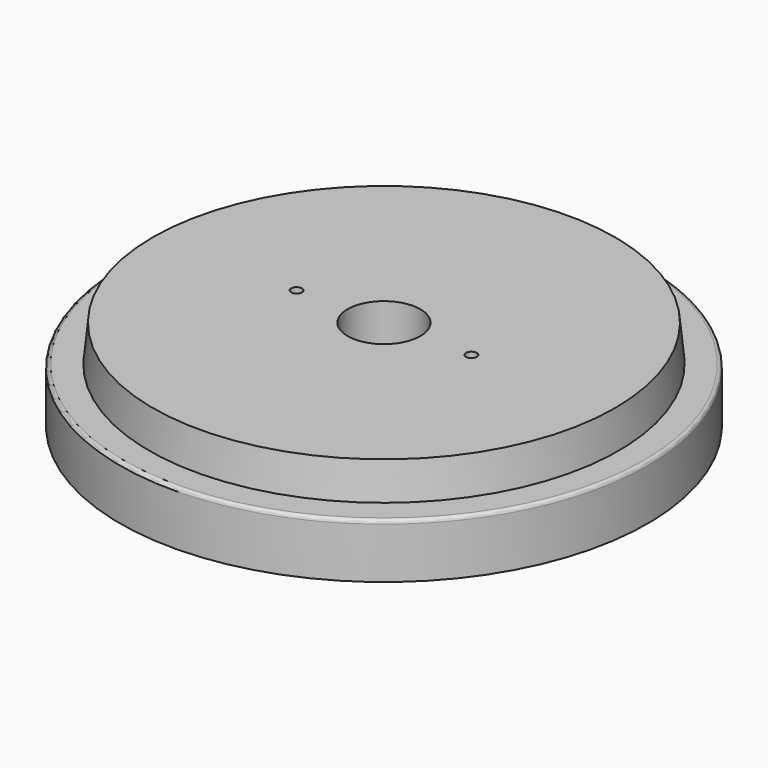
from build123d import *

# Parameters (mm, degrees)
F0_W     = 10
F0_H     = 18.0418604054
F0_H_2   = 25
F0_H_3   = 6.9581395946
F3_R     = 10
F4_DEPTH = 141.6
F5_R     = 1
F6_SIZE2 = 0.99999
F6_SIZE  = 9.99999
F8_D     = 3
F9_D     = 3


# Not quite as in the source:
# - a fillet or chamfer is up to 0.001 mm smaller than in the source, because OpenCascade refuses the exact size


with BuildPart() as f1:
    # F0 (on Front) → F1 (revolve)
    with BuildSketch(Plane.XZ):
        Polygon((-72.5, 15), (-72.5, 0), (0, 0), (0, 25), (-64.5, 25), (-64.5, 15), align=None)
    revolve(axis=Axis((0, 0, 12.5), (0, 0, 1)))

    # F0 (on Front) → F2 (revolve, cut)
    with BuildSketch(Plane.XZ):
        with Locations((5, 34.0209302027)):
            Rectangle(F0_W, F0_H)
        with Locations((5, 12.5)):
            Rectangle(F0_W, F0_H_2)
        with Locations((5, -3.4790697973)):
            Rectangle(F0_W, F0_H_3)
    revolve(axis=Axis((0, 0, 18.0418604054), (0, 0, 1)), mode=Mode.SUBTRACT)

    # F3 (on Front) → F4 (cut)
    with BuildSketch(Plane.XZ):
        Circle(F3_R)
    extrude(amount=-F4_DEPTH, mode=Mode.SUBTRACT)

    # F5
    f5_edges = [f1.edges().sort_by_distance(p)[0] for p in [
        (72.5, 0, 15),
    ]]
    fillet(f5_edges, radius=F5_R)

    # F6 (size 10 and 1 in the source; OpenCascade refuses exactly that, so slightly less here)
    f6_edges = [f1.edges().sort_by_distance(p)[0] for p in [
        (64.5, 0, 25),
    ]]
    chamfer(f6_edges, length=F6_SIZE, length2=F6_SIZE2)

    # F8 (through all)
    with Locations(Plane(origin=(0, 0, 0), x_dir=(1, 0, 0), z_dir=(0, 0, -1))):
        with Locations((24, 0)):
            Hole(F8_D / 2)

    # F9 (through all)
    with Locations(Plane(origin=(0, 0, 0), x_dir=(1, 0, 0), z_dir=(0, 0, -1))):
        with Locations((-24, 0)):
            Hole(F9_D / 2)


solid = f1.part
